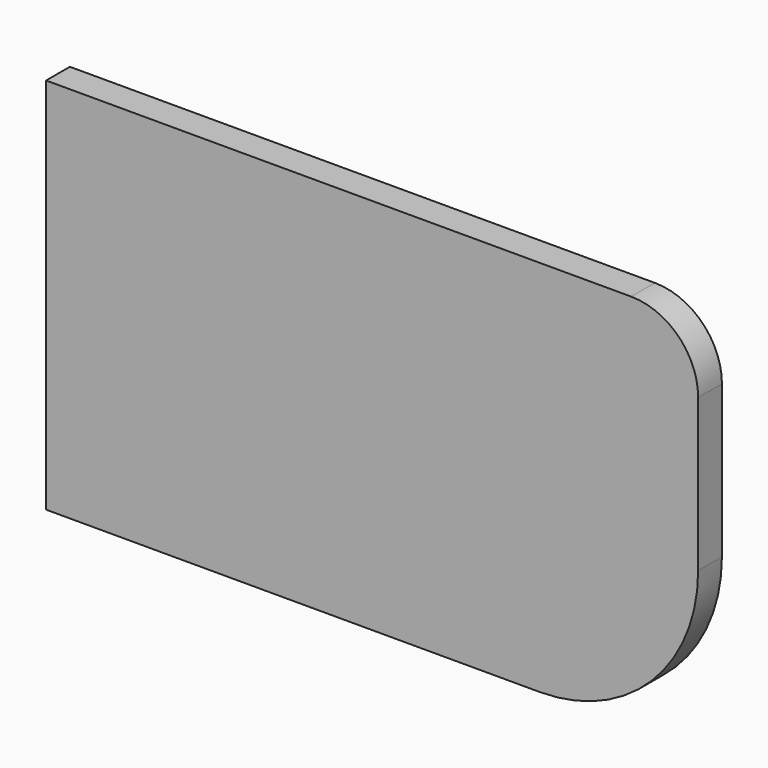
from build123d import *

# Parameters (mm, degrees)
F1_DEPTH = 32.5
F2_DEPTH = 65
F3_DEPTH = 32.5


# Not quite as in the source:
# - a feature names something its author has since deleted; it is built from what else it names


with BuildPart() as f1:
    # F0 (on Front) → F1 (new body, symmetric)
    with BuildSketch(Plane.XZ):
        with BuildLine():
            Line((1900, 0), (0, 0))
            Line((0, 0), (0, -1200))
            Line((0, -1200), (1600, -1200))
            ThreePointArc((1600, -1200), (1953.5533905933, -1053.5533905933), (2100, -700))
            Line((2100, -700), (2100, -200))
            ThreePointArc((2100, -200), (2041.4213562373, -58.5786437627), (1900, 0))
        make_face()
    extrude(amount=F1_DEPTH, both=True)

    # F0 (on Front) → F2 (join)
    with BuildSketch(Plane.XZ):
        with BuildLine():
            Line((-20, -1220), (1600, -1220))
            ThreePointArc((1600, -1220), (1967.695526217, -1067.695526217), (2120, -700))
            Line((2120, -700), (2120, -200))
            ThreePointArc((2120, -200), (2055.563491861, -44.436508139), (1900, 20))
            Line((1900, 20), (-20, 20))
            Line((-20, 20), (-20, -1220))
        make_face()
        with BuildLine():
            Line((0, -1200), (0, 0))
            Line((0, 0), (1900, 0))
            ThreePointArc((1900, 0), (2041.4213562373, -58.5786437627), (2100, -200))
            Line((2100, -200), (2100, -700))
            ThreePointArc((2100, -700), (1953.5533905933, -1053.5533905933), (1600, -1200))
            Line((1600, -1200), (0, -1200))
        make_face(mode=Mode.SUBTRACT)
    extrude(amount=-F2_DEPTH)

    # F0 (on Front) → F3 (join)
    with BuildSketch(Plane.XZ):
        with BuildLine():
            Line((-20, -1220), (1600, -1220))
            ThreePointArc((1600, -1220), (1967.695526217, -1067.695526217), (2120, -700))
            Line((2120, -700), (2120, -200))
            ThreePointArc((2120, -200), (2055.563491861, -44.436508139), (1900, 20))
            Line((1900, 20), (-20, 20))
            Line((-20, 20), (-20, -1220))
        make_face()
        with BuildLine():
            Line((0, -1200), (0, 0))
            Line((0, 0), (1900, 0))
            ThreePointArc((1900, 0), (2041.4213562373, -58.5786437627), (2100, -200))
            Line((2100, -200), (2100, -700))
            ThreePointArc((2100, -700), (1953.5533905933, -1053.5533905933), (1600, -1200))
            Line((1600, -1200), (0, -1200))
        make_face(mode=Mode.SUBTRACT)
    extrude(amount=F3_DEPTH)


solid = f1.part
